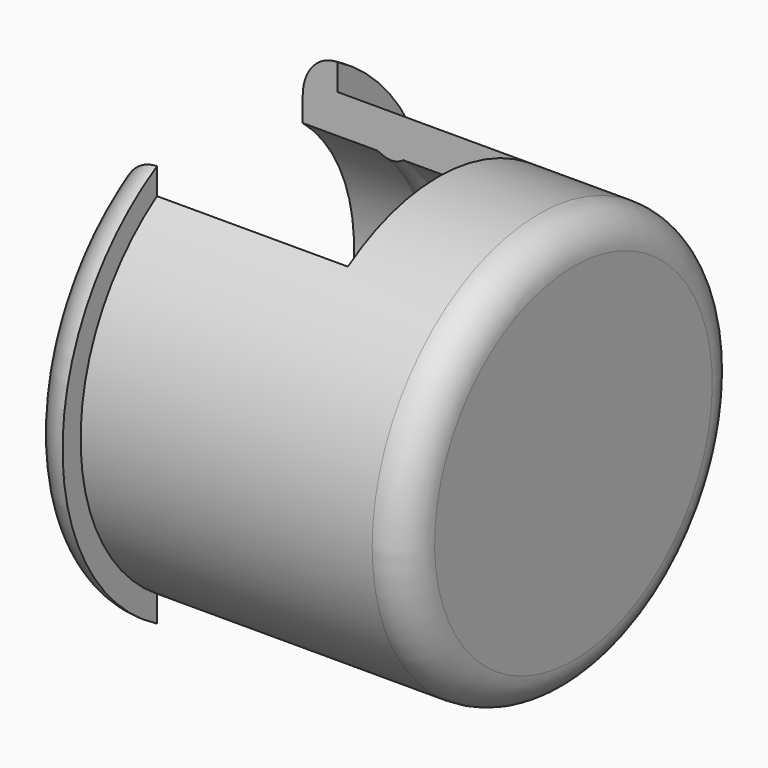
from build123d import *

# Parameters (mm, degrees)
F1_R     = 1.99999
F2_DEPTH = 25
F6_R     = 2


# Not quite as in the source:
# - a fillet or chamfer that OpenCascade refuses, or shapes differently, is made with other operations: its cross-section is extruded or revolved along the edge and cut away or added
# - a fillet or chamfer is up to 0.001 mm smaller than in the source, because OpenCascade refuses the exact size


with BuildPart() as f0:
    # F3 (on Front) → F0 (revolve)
    with BuildSketch(Plane.XZ):
        Polygon((-2, 0), (0, 0), (0, 12), (-18.8, 12), (-18.8, 13.3), (-20.8, 13.3), (-20.8, 10.2), (-16.5, 10.2), (-15, 10.2), (-11.6, 10.2), (-10.1, 10.2), (-2, 10.2), align=None)
        Polygon((-14.9505181851, 9.7), (-15, 10.2), (-16.5, 10.2), align=None)
        Polygon((-10.2909830056, 9.7), (-10.1, 10.2), (-11.6, 10.2), align=None)
    revolve(axis=Axis((-1, 0, 0), (1, 0, 0)))

    # F1 (radius 2 in the source; OpenCascade refuses exactly that, so slightly less here)
    f1_edges = [f0.edges().sort_by_distance(p)[0] for p in [
        (-20.8, 0, -13.3),
    ]]
    fillet(f1_edges, radius=F1_R)

    # F4: fillet of radius 1.5 on 2 edges, made by hand

    # F4_s1 → F4_t2 (revolve, cut)
    with BuildSketch(Plane.XZ):
        with BuildLine():
            ThreePointArc((-16.1707444356, 10.0937530079), (-15.5745304293, 10.0274099354), (-15, 10.2))
            Line((-15, 10.2), (-14.9505181851, 9.7))
            Line((-14.9505181851, 9.7), (-16.1707444356, 10.0937530079))
        make_face()
    revolve(axis=Axis((-14.9505181851, 0, 0), (1, 0, 0)), mode=Mode.SUBTRACT)

    # F4_s3 → F4_t4 (revolve, cut)
    with BuildSketch(Plane.XZ):
        with BuildLine():
            ThreePointArc((-11.3639501712, 10.1098369884), (-10.721986782, 10.0148974609), (-10.1, 10.2))
            Line((-10.1, 10.2), (-10.2909830056, 9.7))
            Line((-10.2909830056, 9.7), (-11.3639501712, 10.1098369884))
        make_face()
    revolve(axis=Axis((-10.2909830056, 0, 0), (1, 0, 0)), mode=Mode.SUBTRACT)

    # F5 (on Top) → F2 (cut, symmetric)
    with BuildSketch(Plane.XY):
        Polygon((-7.8, 6.5), (-30.9797403524, 6.5), (-30.8855128417, -6.5), (-7.8, -6.5), align=None)
    extrude(amount=F2_DEPTH, both=True, mode=Mode.SUBTRACT)

    # F6
    f6_edges = [f0.edges().sort_by_distance(p)[0] for p in [
        (0, 0, -12),
    ]]
    fillet(f6_edges, radius=F6_R)


solid = f0.part
